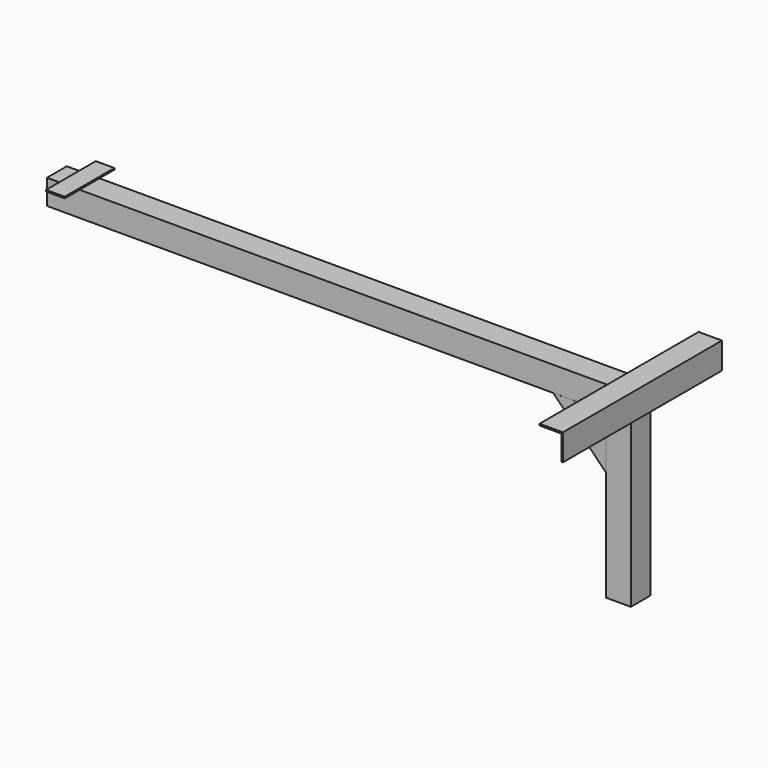
from build123d import *

# Parameters (mm, degrees)
F0_W      = 50.8
F0_H      = 406.4
F1_DEPTH  = 6.35
F2_W      = 6.35
F2_H      = 406.4
F3_DEPTH  = 50.8
F4_DEPTH  = 3.048
F5_DEPTH  = 3.048
F6_W      = 1149.35
F6_H      = 50.8
F7_DEPTH  = 50.8
F8_W      = 38.1
F8_H      = 50.8
F8_H_2    = 38.1
F9_DEPTH  = 3.048
F10_W     = 50.8
F10_H     = 50.8
F11_DEPTH = 333.375
F13_DEPTH = 50.8


# Not quite as in the source:
# - a feature names something its author has since deleted; it is built from what else it names


with BuildPart() as f1:
    # F0 (on Top) → F1 (new body)
    with BuildSketch(Plane.XY):
        Rectangle(F0_W, F0_H)
    extrude(amount=F1_DEPTH)

    # F2 (on face) → F3 (join)
    with BuildSketch(Plane(origin=(0, 0, 0), x_dir=(1, 0, 0), z_dir=(0, 0, -1))):
        with Locations((22.225, 0)):
            Rectangle(F2_W, F2_H)
    extrude(amount=F3_DEPTH)

    # F4 (cut): a face of the model
    f4_faces = [f1.faces().sort_by_distance(p)[0] for p in [
        (25.4, 0, -22.225),
    ]]
    extrude(f4_faces, amount=-F4_DEPTH, mode=Mode.SUBTRACT)

    # F5 (cut): a face of the model
    f5_faces = [f1.faces().sort_by_distance(p)[0] for p in [
        (-1.524, 0, 6.35),
    ]]
    extrude(f5_faces, amount=-F5_DEPTH, mode=Mode.SUBTRACT)

    # F6 (on face) → F7 (join)
    with BuildSketch(Plane(origin=(0, 0, 0), x_dir=(1, 0, 0), z_dir=(0, 0, -1))):
        Polygon((19.05, -25.4), (19.05, 0), (19.05, 25.4), (-25.4, 25.4), (-25.4, -25.4), align=None)
        with Locations((-600.075, 0)):
            Rectangle(F6_W, F6_H)
    extrude(amount=F7_DEPTH)

    # F8 (on face) → F9 (join)
    with BuildSketch(Plane.XY):
        with Locations((-1126.998, 0)):
            Rectangle(F8_W, F8_H)
        with Locations((-1126.998, 44.45)):
            Rectangle(F8_W, F8_H_2)
        with Locations((-1126.998, -44.45)):
            Rectangle(F8_W, F8_H_2)
    extrude(amount=F9_DEPTH)

    # F10 (on face) → F11 (join)
    with BuildSketch(Plane(origin=(0, 0, -50.8), x_dir=(1, 0, 0), z_dir=(0, 0, -1))):
        with Locations((-6.35, 0)):
            Rectangle(F10_W, F10_H)
    extrude(amount=F11_DEPTH)


with BuildPart() as f13:
    # F12 (on face) → F13 (new body)
    with BuildSketch(Plane.XZ.offset(25.4)):
        Polygon((-67.7644877579, -50.8934632736), (-139.7, -50.8), (-31.75, -158.75), (-31.75, -86.9079510314), (-49.8039755157, -68.8539755157), align=None)
    extrude(amount=-F13_DEPTH)


solid = Compound([f1.part, f13.part])
